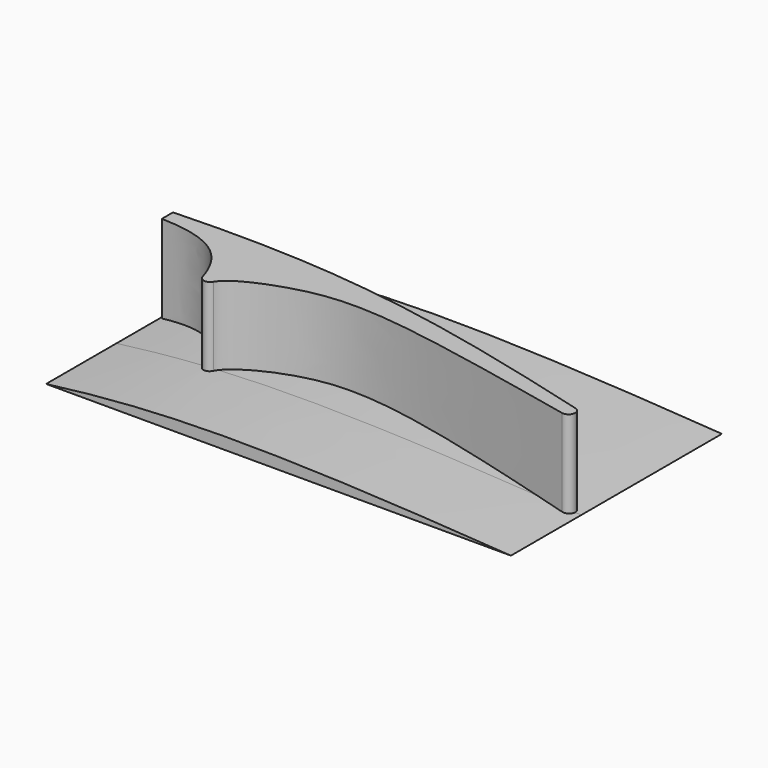
from build123d import *

# Parameters (mm, degrees)
F2_DEPTH      = 25.4
F2_DEPTH_BACK = 50.8
F3_DEPTH      = 25.4


with BuildPart() as f2:
    # F1 (on Front) → F2 (new body, two sides)
    with BuildSketch(Plane.XZ) as f2_sk:
        with BuildLine():
            add(Edge.make_bspline(
                [(-66.493101418, 0), (-31.6023416817, 4.5892358758), (0, 4.5892358758), (67.7957311273, 0)],
                knots=[0, 0, 0, 0, 134.2888325453, 134.2888325453, 134.2888325453, 134.2888325453], degree=3))
            Line((-66.493101418, 0), (67.7957311273, 0))
        make_face()
    extrude(amount=F2_DEPTH)
    extrude(f2_sk.sketch, amount=-F2_DEPTH_BACK)

    # F0 (on Top) → F3 (join)
    with BuildSketch(Plane.XY):
        with BuildLine():
            add(Edge.make_bspline(
                [(-66.0190582275, 15.8042479306), (-50.882216543, 15.443845652), (-44.3860767732, 10.0356803936), (-41.1722754867, -0.5532574777)],
                knots=[0, 0, 0, 0, 29.7477830393, 29.7477830393, 29.7477830393, 29.7477830393], degree=3))
            ThreePointArc((-41.1722754867, -0.5532574777), (-39.5395729632, -1.8954823631), (-37.6727509093, -0.9043917556))
            add(Edge.make_bspline(
                [(-37.6727509093, -0.9043917556), (-35.9554500646, 2.279277761), (-11.7834584129, 13.3395817627), (10.1645017819, 9.6475739081), (63.7337581556, -1.8624929201)],
                knots=[0, 0, 0, 0, 0.3222291325, 1, 1, 1, 1], degree=3))
            ThreePointArc((63.7337581556, -1.8624929201), (65.9847645302, -0.4510784554), (64.6355761504, 1.8377664946))
            add(Edge.make_bspline(
                [(-66.0190582275, 19.8427634791), (-18.4567762815, 21.7484285157), (11.260919046, 16.4069097143), (64.6355761504, 1.8377664946)],
                knots=[0, 0, 0, 0, 131.8893983641, 131.8893983641, 131.8893983641, 131.8893983641], degree=3))
            Line((-66.0190582275, 19.8427634791), (-66.0190582275, 15.8042479306))
        make_face()
    extrude(amount=F3_DEPTH)


solid = f2.part
